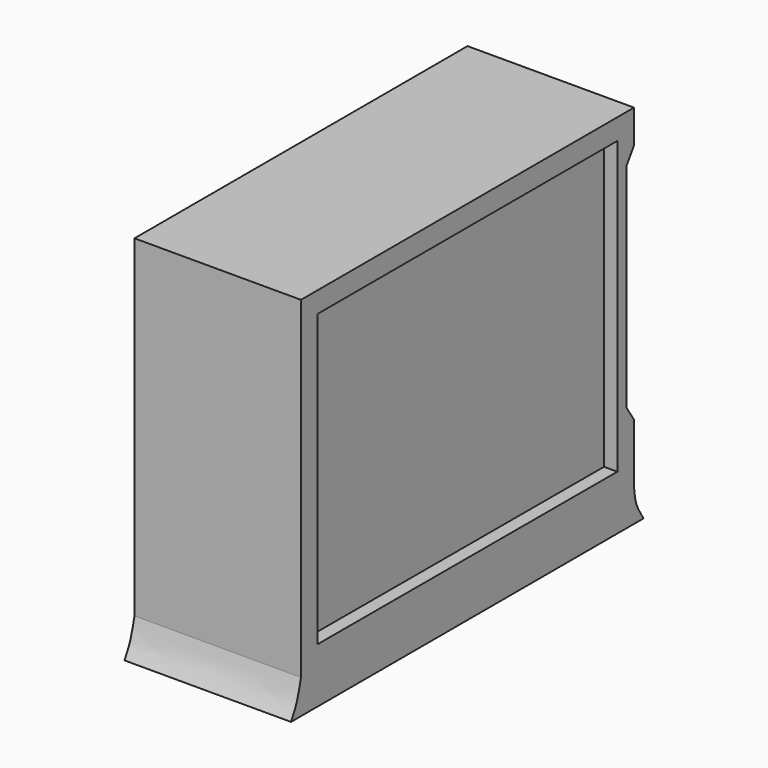
from build123d import *

# Parameters (mm, degrees)
F1_DEPTH = 50.8
F2_DEPTH = 2.54
F5_START = 43.18
F5_DEPTH = 1.016
F6_START = -61.722
F4_W     = 5.842
F4_H     = 12.7
F4_W_2   = 3.81
F4_H_2   = 38.1
F6_DEPTH = 1.524


# Not quite as in the source:
# - a feature of the source that left no trace in its solid (it failed there, or was rolled back) is left out


with BuildPart() as f1:
    # F0 (on Right) → F1 (new body)
    with BuildSketch(Plane.YZ):
        Polygon((-61.698825866, 55.9749106665), (-61.698825866, -45.4361034706), (65.301174134, -45.5878325482), (65.301174134, -27.8078325482), (62.494367, -23.5736580464), (62.494367, 41.5807361647), (65.301174134, 45.8149106665), (65.301174134, 55.9749106665), align=None)
        Polygon((-55.3488239149, -39.093683444), (-55.3488239149, 49.6249087155), (58.951172183, 49.6249087155), (58.951172183, -39.2302396091), align=None, mode=Mode.SUBTRACT)
        with BuildLine():
            Line((65.301174134, -45.5878325482), (-61.698825866, -45.4361034706))
            add(Edge.make_bspline(
                [(-65.5058175325, -55.8386668563), (-64.7629052579, -54.5340589091), (-63.1453130575, -51.6934494428), (-62.2064804259, -47.6321617795), (-61.698825866, -45.4361034706)],
                knots=[0, 0, 0, 0, 0.4592704357, 1, 1, 1, 1], degree=3))
            Line((-65.5058175325, -55.8386668563), (68.9185634255, -55.8386668563))
            add(Edge.make_bspline(
                [(68.9185634255, -55.8386668563), (67.8020531364, -54.0848642317), (65.6584922314, -50.7307193347), (65.4183999928, -47.2370915893), (65.301174134, -45.5878325482)],
                knots=[0, 0, 0, 0, 0.5226245331, 1, 1, 1, 1], degree=3))
        make_face()
    extrude(amount=F1_DEPTH)

    # F0 (on Right) → F2 (join)
    with BuildSketch(Plane.YZ):
        Polygon((58.951172183, 49.6249087155), (-55.3488239149, 49.6249087155), (-55.3488239149, -39.093683444), (58.951172183, -39.2302396091), align=None)
    extrude(amount=F2_DEPTH)

    # F2_face (on face) → F5 (join)
    with BuildSketch(Plane(origin=(2.54, 1.8158237937, 5.2314648434), x_dir=(0, 1, 0), z_dir=(1, 0, 0)).offset(F5_START)):
        Polygon((57.1353483893, -44.4617044525), (57.1353483893, 44.3934438721), (-57.1646477086, 44.3934438721), (-57.1646477086, -44.3251482873), align=None)
    extrude(amount=F5_DEPTH)

    # F4 (on Front) → F6 (join)
    with BuildSketch(Plane.XZ.offset(F6_START)):
        with BuildLine():
            Line((39.7206060588, -9.1834223449), (39.7206060588, 28.9165776551))
            Line((39.7206060588, 28.9165776551), (33.9717225262, 28.9165776551))
            ThreePointArc((33.9717225262, 28.9165776551), (31.8466060588, 27.6465776551), (29.7214895914, 28.9165776551))
            Line((29.7214895914, 28.9165776551), (22.506811127, 28.9165776551))
            ThreePointArc((22.506811127, 28.9165776551), (20.3816946596, 27.6465776551), (18.2565781922, 28.9165776551))
            Line((18.2565781922, 28.9165776551), (11.7806060588, 28.9165776551))
            Line((11.7806060588, 28.9165776551), (11.7806060588, -9.1834223449))
            Line((11.7806060588, -9.1834223449), (39.7206060588, -9.1834223449))
        make_face()
        with Locations((19.1466060588, 0.9765776551)):
            Rectangle(F4_W, F4_H, mode=Mode.SUBTRACT)
        with Locations((32.3546060588, 0.9765776551)):
            Rectangle(F4_W, F4_H, mode=Mode.SUBTRACT)
        with Locations((19.1466060588, 18.1998224765)):
            Rectangle(F4_W, F4_H, mode=Mode.SUBTRACT)
        with Locations((32.3546060588, 18.2028314263)):
            Rectangle(F4_W, F4_H, mode=Mode.SUBTRACT)
        with BuildLine():
            Line((33.9717225262, 28.9165776551), (39.7206060588, 28.9165776551))
            ThreePointArc((39.7206060588, 28.9165776551), (38.6315341138, 32.4725776551), (35.7378860588, 34.8088170767))
            Line((35.7378860588, 34.8088170767), (15.7633260588, 34.8088170767))
            ThreePointArc((15.7633260588, 34.8088170767), (12.8696780038, 32.4725776551), (11.7806060588, 28.9165776551))
            Line((11.7806060588, 28.9165776551), (18.2565781922, 28.9165776551))
            ThreePointArc((18.2565781922, 28.9165776551), (19.7923463058, 32.3995002004), (22.7946946596, 30.0595776551))
            ThreePointArc((22.7946946596, 30.0595776551), (22.7216172049, 29.4702293013), (22.506811127, 28.9165776551))
            Line((22.506811127, 28.9165776551), (29.7214895914, 28.9165776551))
            ThreePointArc((29.7214895914, 28.9165776551), (31.2572577051, 32.3995002004), (34.2596060588, 30.0595776551))
            ThreePointArc((34.2596060588, 30.0595776551), (34.1865286041, 29.4702293013), (33.9717225262, 28.9165776551))
        make_face()
        with Locations((7.3356060588, 9.8665776551)):
            Rectangle(F4_W_2, F4_H_2)
    extrude(amount=-F6_DEPTH)


solid = f1.part
